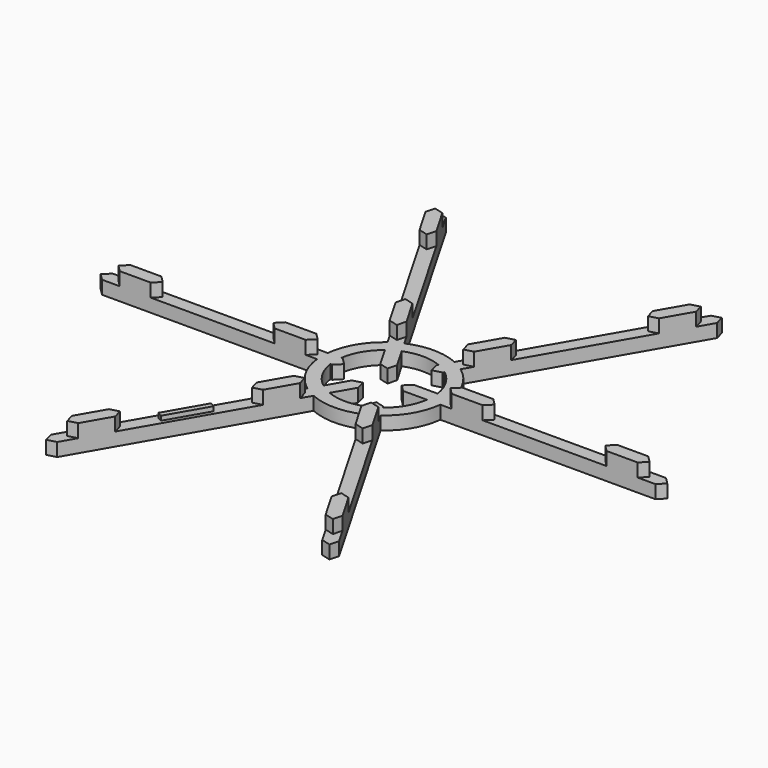
from build123d import *

# Parameters (mm, degrees)
F1_DEPTH = 3
F4_DEPTH = 3
F5_COUNT = 3
F5_ANGLE = 240
F7_DEPTH = 1
F8_R     = 14
F8_R_2   = 11
F9_DEPTH = 3


# Not quite as in the source:
# - a feature names something its author has since deleted; it is built from what else it names


with BuildPart() as f1:
    # F0 (on Top) → F1 (new body)
    with BuildSketch(Plane.XY):
        Polygon((-2, -3.4641016151), (-4.0490381057, -4.0131397208), (-32.5490381057, -53.3765877365), (-32, -55.4256258422), (-29.9509618943, -54.8765877365), (-1.4509618943, -5.5131397208), align=None)
    extrude(amount=F1_DEPTH)

    # F3 (on face) → F4, piece 2 (join)
    with BuildSketch(Plane.XY.offset(3)):
        Polygon((-27.0490381057, -43.8503082949), (-30.5490381057, -49.9124861214), (-30, -51.9615242271), (-27.9509618943, -51.4124861214), (-24.4509618943, -45.3503082949), (-25, -43.3012701892), align=None)
        Polygon((-9.5490381057, -13.5394191624), (-13.0490381057, -19.6015969889), (-12.5, -21.6506350946), (-10.4509618943, -21.1015969889), (-6.9509618943, -15.0394191624), (-7.5, -12.9903810568), align=None)
    extrude(amount=F4_DEPTH)


with BuildPart() as f1b:
    # F0 (on Top) → F1, piece 2 (new body)
    with BuildSketch(Plane.XY):
        Polygon((-10.5, 1.5), (-62.5, 1.5), (-64, 0), (-62.5, -1.5), (-10.5, -1.5), (-9, 0), align=None)
    extrude(amount=F1_DEPTH)

    # F3 (on face) → F4 (join)
    with BuildSketch(Plane.XY.offset(3)):
        Polygon((-51.5, 1.5), (-58.5, 1.5), (-60, 0), (-58.5, -1.5), (-51.5, -1.5), (-50, 0), align=None)
        Polygon((-16.5, 1.5), (-23.5, 1.5), (-25, 0), (-23.5, -1.5), (-16.5, -1.5), (-15, 0), align=None)
    extrude(amount=F4_DEPTH)


with BuildPart() as f5_1:
    # F5: instance of F1
    add(f1.part.rotate(Axis((0, 0, 0.1916177571), (0, 0, -1)), 1 * F5_ANGLE / (F5_COUNT - 1)))


with BuildPart() as f5_2:
    # F5: instance of F1
    add(f1.part.rotate(Axis((0, 0, 0.1916177571), (0, 0, -1)), 2 * F5_ANGLE / (F5_COUNT - 1)))


with BuildPart() as f5_3:
    # F5: instance of F1b
    add(f1b.part.rotate(Axis((0, 0, 0.1916177571), (0, 0, -1)), 1 * F5_ANGLE / (F5_COUNT - 1)))


with BuildPart() as f5_4:
    # F5: instance of F1b
    add(f1b.part.rotate(Axis((0, 0, 0.1916177571), (0, 0, -1)), 2 * F5_ANGLE / (F5_COUNT - 1)))


with BuildPart() as f1_1:
    add(f1.part)

    # F6 (on face) → F7 (join)
    with BuildSketch(Plane.XY.offset(3)):
        Polygon((-15.7303847577, -28.445825623), (-16.7696152423, -27.845825623), (-21.7696152423, -36.5060796608), (-20.7303847577, -37.1060796608), align=None)
    extrude(amount=F7_DEPTH)

    add(f1b.part)  # F9 merges F1b

    add(f5_1.part)  # F9 merges F5_1

    add(f5_2.part)  # F9 merges F5_2

    add(f5_3.part)  # F9 merges F5_3

    add(f5_4.part)  # F9 merges F5_4
    # F8 (on Top) → F9 (join)
    with BuildSketch(Plane.XY):
        Circle(F8_R)
        Circle(F8_R_2, mode=Mode.SUBTRACT)
    extrude(amount=F9_DEPTH)


solid = f1_1.part
